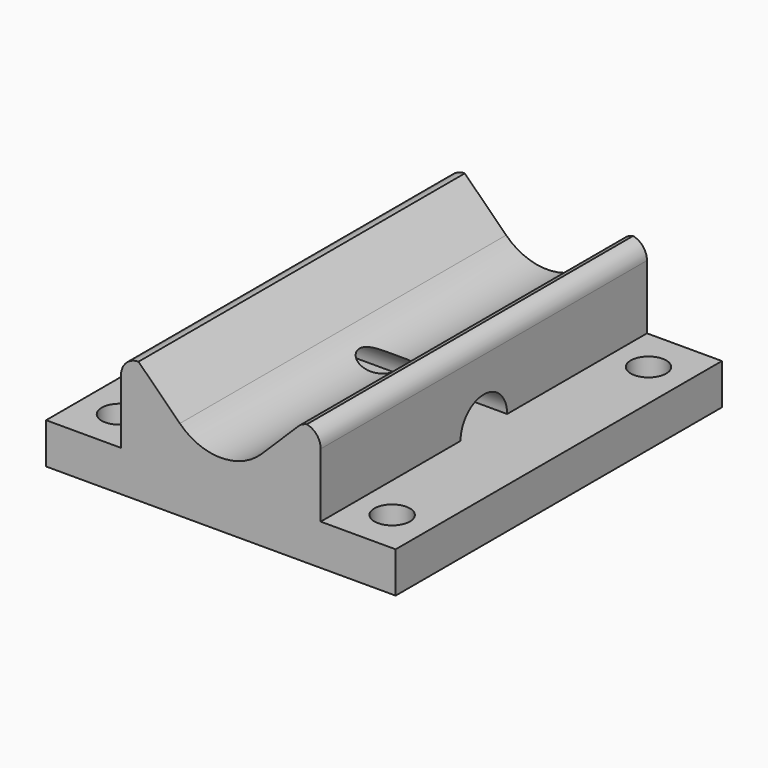
from build123d import *

# Parameters (mm, degrees)
F0_W         = 30
F0_H         = 35
F1_DEPTH     = 13
F2_W         = 3.9074438825
F2_H         = 9.5
F3_DEPTH     = 35.001
F4_W         = 2.524356873
F4_H         = 7
F5_DEPTH     = 35.001
F6_R         = 5
F8_DEPTH     = 30.001
F9_R         = 1.5246036127
F10_DEPTH    = 10.501
F11_T1_DEPTH = 42.5
F11_T3_DEPTH = 38.085325067


# Not quite as in the source:
# - a fillet or chamfer that OpenCascade refuses, or shapes differently, is made with other operations: its cross-section is extruded or revolved along the edge and cut away or added


with BuildPart() as f1:
    # F0 (on Top) → F1 (new body)
    with BuildSketch(Plane.XY):
        with Locations((15, 17.5)):
            Rectangle(F0_W, F0_H)
    extrude(amount=F1_DEPTH)

    # F2 (on face) → F3 (cut, through all)
    with BuildSketch(Plane.XZ):
        with Locations((1.9537219413, 8.25)):
            Rectangle(F2_W, F2_H)
        Polygon((15, 13), (5.4074438825, 13), (15, 3.5), (24.5925561175, 13), align=None)
        with Locations((28.0462780587, 8.25)):
            Rectangle(F2_W, F2_H)
    extrude(amount=-F3_DEPTH, mode=Mode.SUBTRACT)

    # F4 (on face) → F5 (cut, through all)
    with BuildSketch(Plane.XZ):
        Polygon((6.4318007555, 10.5), (7.9318007555, 10.5), (5.4074438825, 13), (3.9074438825, 13), (3.9074438825, 10.5), align=None)
        Polygon((23.5681992445, 10.5), (26.0925561175, 10.5), (26.0925561175, 13), (24.5925561175, 13), (22.0681992445, 10.5), align=None)
        with Locations((5.169622319, 7)):
            Rectangle(F4_W, F4_H)
        with Locations((24.830377681, 7)):
            Rectangle(F4_W, F4_H)
    extrude(amount=-F5_DEPTH, mode=Mode.SUBTRACT)

    # F6
    f6_edges = [f1.edges().sort_by_distance(p)[0] for p in [
        (15, 17.5, 3.5),
    ]]
    fillet(f6_edges, radius=F6_R)

    # F7 (on face) → F8 (cut, through all)
    with BuildSketch(Plane(origin=(0, 0, 0), x_dir=(0, -1, 0), z_dir=(-1, 0, 0))):
        with BuildLine():
            ThreePointArc((-15, 3.5), (-17.5, 6), (-20, 3.5))
            Line((-20, 3.5), (-15, 3.5))
        make_face()
    extrude(amount=-F8_DEPTH, mode=Mode.SUBTRACT)

    # F9 (on face) → F10 (cut, through all)
    with BuildSketch(Plane(origin=(0, 0, 0), x_dir=(1, 0, 0), z_dir=(0, 0, -1))):
        with Locations((3.3, -3.75)):
            Circle(F9_R)
        with Locations((26.7, -3.75)):
            Circle(F9_R)
        with Locations((3.3, -31.25)):
            Circle(F9_R)
        with Locations((26.7, -31.25)):
            Circle(F9_R)
    extrude(amount=-F10_DEPTH, mode=Mode.SUBTRACT)

    # F11: fillet of radius 1.5 on 3 edges, made by hand

    # F11_s2 → F11_t1 (cut)
    with BuildSketch(Plane.XZ.offset(-38.75)):
        with BuildLine():
            ThreePointArc((7.9318007555, 10.5), (6.8711405838, 10.0606601718), (6.4318007555, 9))
            Line((6.4318007555, 9), (6.4318007555, 10.5))
            Line((6.4318007555, 10.5), (7.9318007555, 10.5))
        make_face()
        with BuildLine():
            ThreePointArc((22.0681992445, 10.5), (23.1288594162, 10.0606601718), (23.5681992445, 9))
            Line((23.5681992445, 9), (23.5681992445, 10.5))
            Line((23.5681992445, 10.5), (22.0681992445, 10.5))
        make_face()
    extrude(amount=F11_T1_DEPTH, mode=Mode.SUBTRACT)

    # F11_s4 → F11_t3 (cut)
    with BuildSketch(Plane.XZ.offset(-36.5426625335)):
        with BuildLine():
            ThreePointArc((21.6297583139, 10.0657894737), (22.1145998252, 10.3872065835), (22.6852642579, 10.5))
            Line((22.6852642579, 10.5), (22.0681992445, 10.5))
            Line((22.0681992445, 10.5), (21.6297583139, 10.0657894737))
        make_face()
    extrude(amount=F11_T3_DEPTH, mode=Mode.SUBTRACT)


solid = f1.part
